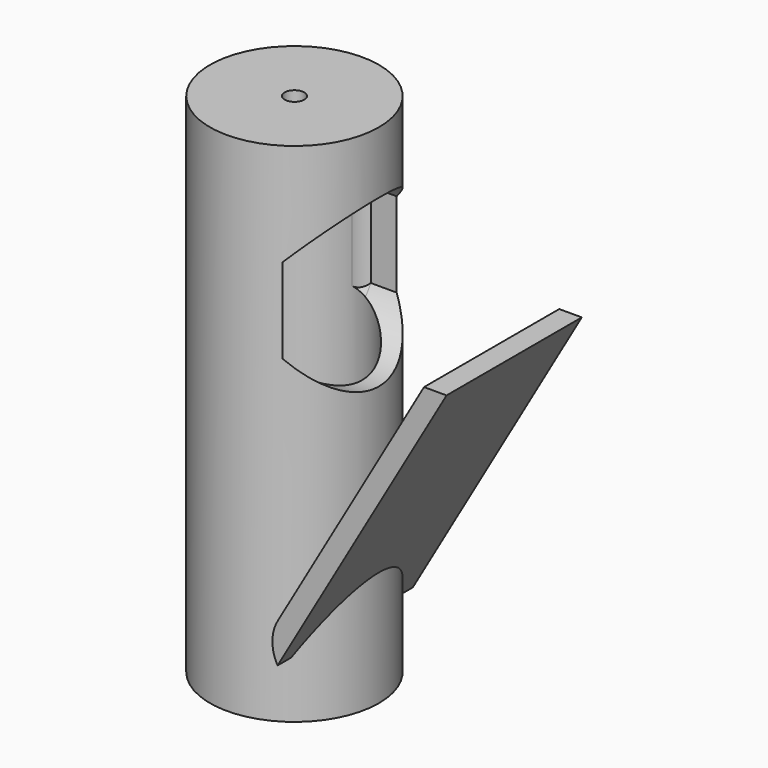
from build123d import *

# Parameters (mm, degrees)
F0_R         = 15
F0_R_2       = 12
F1_DEPTH     = 90
F0_R_3       = 1.75
F2_DEPTH     = 8
F5_DEPTH     = 11.6
F6_T4_DEPTH  = 32.7089830992
F6_S5_R      = 14.75
F6_T6_DEPTH  = 18
F6_T10_DEPTH = 32.7089830992
F6_S11_R     = 14.75
F6_T12_DEPTH = 18
F9_DEPTH     = 30
F10_T1_DEPTH = 70.2065483844
F11_DEPTH    = 103.2


# Not quite as in the source:
# - a fillet or chamfer that OpenCascade refuses, or shapes differently, is made with other operations: its cross-section is extruded or revolved along the edge and cut away or added


with BuildPart() as f1:
    # F0 (on Top) → F1 (new body)
    with BuildSketch(Plane.XY):
        Circle(F0_R)
        Circle(F0_R_2, mode=Mode.SUBTRACT)
    extrude(amount=-F1_DEPTH)

    # F0 (on Top) → F2 (join)
    with BuildSketch(Plane.XY):
        Circle(F0_R_2)
        Circle(F0_R_3, mode=Mode.SUBTRACT)
    extrude(amount=-F2_DEPTH)

    # F4 (on offset) → F5 (cut)
    with BuildSketch(Plane.YZ.offset(15)):
        with BuildLine():
            Line((12.688, -33.271778779), (12.688, -18.228221221))
            ThreePointArc((12.688, -18.228221221), (0, -11), (-12.688, -18.228221221))
            Line((-12.688, -18.228221221), (-12.688, -33.271778779))
            ThreePointArc((-12.688, -33.271778779), (0, -40.5), (12.688, -33.271778779))
        make_face()
    extrude(amount=-F5_DEPTH, mode=Mode.SUBTRACT)

    # F6: fillet of radius 5 on 2 edges, made by hand


with BuildPart() as f6_tool2:
    # F6_s3 → F6_t4 (new body)
    with BuildSketch(Plane.XY.offset(-42.1044915496)):
        with BuildLine():
            ThreePointArc((3.4, -12.688), (2.0464541168, -12.1286761902), (0.588907604, -11.9855407819))
            ThreePointArc((0.588907604, -11.9855407819), (2.0086800902, -11.8306890879), (3.4, -11.5082579047))
            Line((3.4, -11.5082579047), (3.4, -12.688))
        make_face()
    extrude(amount=F6_T4_DEPTH)

    # F6_s5 → F6_t6 (intersect, symmetric)
    with BuildSketch(Plane.YZ.offset(2)):
        with Locations((0, -25.75)):
            Circle(F6_S5_R)
    extrude(amount=F6_T6_DEPTH, both=True, mode=Mode.INTERSECT)


with BuildPart() as f1_1:
    add(f1.part)

    # F6_t1: cut F6_tool2
    add(f6_tool2.part, mode=Mode.SUBTRACT)


with BuildPart() as f6_tool8:
    # F6_s9 → F6_t10 (new body)
    with BuildSketch(Plane.XY.offset(-42.1044915496)):
        with BuildLine():
            ThreePointArc((0.588907604, 11.9855407819), (2.0464541168, 12.1286761902), (3.4, 12.688))
            Line((3.4, 12.688), (3.4, 11.5082579047))
            ThreePointArc((3.4, 11.5082579047), (2.0086800902, 11.8306890879), (0.588907604, 11.9855407819))
        make_face()
    extrude(amount=F6_T10_DEPTH)

    # F6_s11 → F6_t12 (intersect, symmetric)
    with BuildSketch(Plane.YZ.offset(2)):
        with Locations((0, -25.75)):
            Circle(F6_S11_R)
    extrude(amount=F6_T12_DEPTH, both=True, mode=Mode.INTERSECT)


with BuildPart() as f1_2:
    add(f1_1.part)

    # F6_t7: cut F6_tool8
    add(f6_tool8.part, mode=Mode.SUBTRACT)


with BuildPart() as f9:
    # F8 (on offset) → F9 (new body)
    with BuildSketch(Plane.XZ.offset(15)):
        Polygon((9, -79.9615242271), (39, -28), (35, -28), (5, -79.9615242271), align=None)
    extrude(amount=-F9_DEPTH)

    # F10: fillet of radius 7 on 1 edges, made by hand

    # F10_s2 → F10_t1 (cut)
    with BuildSketch(Plane.XZ.offset(-35.1032741922)):
        with BuildLine():
            ThreePointArc((9.0206548384, -72.9975457672), (8.0828634538, -76.4767841818), (9, -79.9615242271))
            Line((9, -79.9615242271), (5, -79.9615242271))
            Line((5, -79.9615242271), (9.0206548384, -72.9975457672))
        make_face()
    extrude(amount=F10_T1_DEPTH, mode=Mode.SUBTRACT)

    # F0 (on Top) → F11 (cut)
    with BuildSketch(Plane.XY):
        Circle(F0_R)
        Circle(F0_R_2, mode=Mode.SUBTRACT)
        Circle(F0_R_2)
        Circle(F0_R_3, mode=Mode.SUBTRACT)
    extrude(amount=-F11_DEPTH, mode=Mode.SUBTRACT)


solid = Compound([f1_2.part, f9.part])
